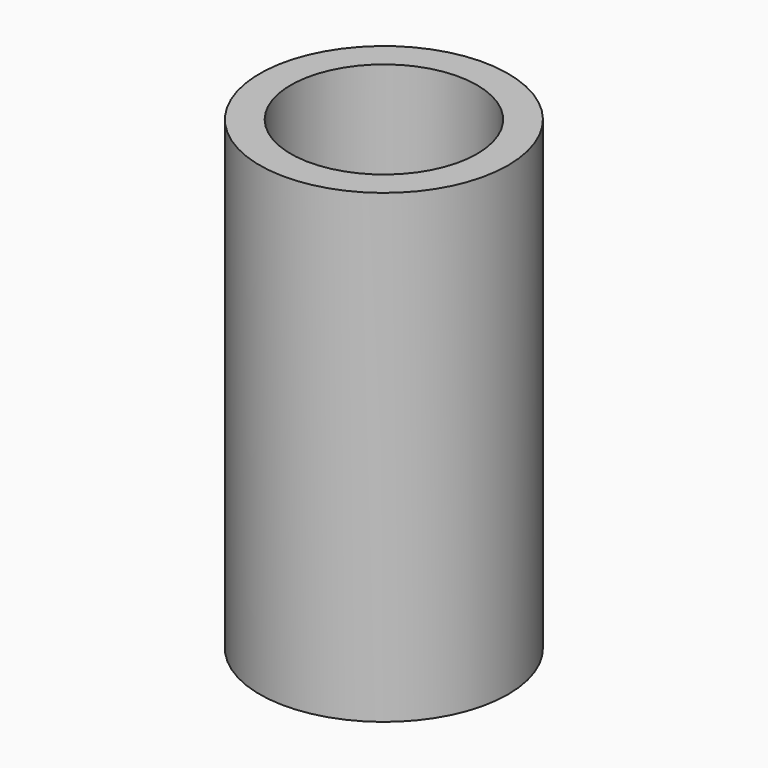
from build123d import *

# Parameters (mm, degrees)
F0_R     = 8
F0_R_2   = 6
F1_DEPTH = 30


# Not quite as in the source:
# - a feature names something its author has since deleted; it is built from what else it names


with BuildPart() as f1:
    # F0 (on Top) → F1 (new body)
    with BuildSketch(Plane.XY):
        Circle(F0_R)
        Circle(F0_R_2, mode=Mode.SUBTRACT)
    extrude(amount=F1_DEPTH)


solid = f1.part
